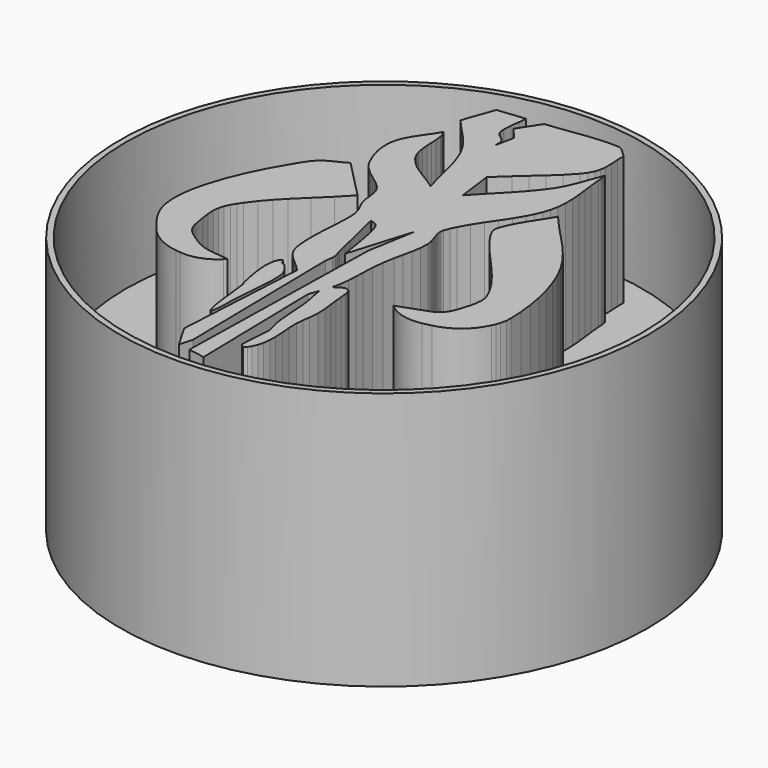
from build123d import *

# Parameters (mm, degrees)
F1_R     = 28.575
F2_DEPTH = 27.94
F0_R     = 27.94
F3_DEPTH = 13.97


# Not quite as in the source:
# - ends of sketch curves that miss each other by under 0.0002 mm in the source are joined


with BuildPart() as f2:
    # F1 (on face) → F2 (new body)
    with BuildSketch(Plane.XY):
        with Locations((1.0160021484, 3.1383140235)):
            Circle(F1_R)
    extrude(amount=-F2_DEPTH)

    # F0 (on Top) → F3 (cut)
    with BuildSketch(Plane.XY):
        with Locations((1.0160021484, 3.1383140235)):
            Circle(F0_R)
        Polygon((-3.3095653584, -5.6137892885), (-3.1695097584, -5.4395960885), (-3.0529237584, -5.4829538885), (-3.0004219584, -5.5103858885), (-2.9673765584, -5.5440408885), (-2.9427639584, -5.5983460885), (-2.9302163584, -5.6597632885), (-2.9131729584, -5.7589248885), (-2.8898557584, -5.8141190885), (-2.8479203584, -5.8575022885), (-2.7512733584, -5.9104104885), (-2.5523405584, -5.9840196885), (-2.5061633584, -6.0104102885), (-2.4849035584, -6.0263360885), (-2.4798235584, -6.0306286885), (-2.4773343584, -6.0328130885), (-2.4760897584, -6.0339306885), (-2.4754801584, -6.0344894885), (-2.4730163584, -6.0367246885), (-2.4632119584, -6.0456654885), (-2.4242229584, -6.0817588885), (-2.2726103584, -6.2308822885), (-1.9922197584, -6.5571706885), (-1.7587429584, -6.9181808885), (-1.5875723584, -7.3190944885), (-1.4959037584, -7.7449508885), (-1.4564575584, -8.7470316885), (-1.5075115584, -9.7528970885), (-1.5761169584, -10.7580258885), (-1.7809679584, -13.4732858885), (-1.8152833584, -14.2048566885), (-1.8169851584, -14.9385864885), (-1.8529515584, -15.6699794885), (-1.9431723584, -16.2117868885), (-1.9748207584, -16.3335290885), (-2.0227759584, -16.4506738885), (-2.0391081584, -16.4671838885), (-2.0507159584, -16.4732036885), (-2.0637969584, -16.4748800885), (-2.0751253584, -16.4723146885), (-2.0914321584, -16.4626372885), (-2.1228773584, -16.4262898885), (-2.1991789584, -16.2593356885), (-2.3008551584, -15.9096792885), (-2.3766995584, -15.5528854885), (-2.5239687584, -14.6005886885), (-2.6334681584, -13.6423736885), (-2.8588677584, -11.7314300885), (-2.9211739584, -11.2544434885), (-2.9539399584, -11.0161660885), (-2.9707801584, -10.8971162885), (-2.9752505584, -10.8818762885), (-2.9848009584, -10.8691762885), (-3.0330101584, -10.8370960885), (-3.0537111584, -10.8222878885), (-3.0650903584, -10.8089274885), (-3.0688241584, -10.8010026885), (-3.0700179584, -10.7968116885), (-3.0702465584, -10.7957448885), (-3.0703227584, -10.7954908885), (-3.0705259584, -10.7944240885), (-3.0713387584, -10.7901314885), (-3.0746661584, -10.7730372885), (-3.0882551584, -10.7046604885), (-3.1452781584, -10.4317374885), (-3.3700173584, -9.3393850885), (-3.4978301584, -8.5924472885), (-3.5894733584, -7.8403786885), (-3.6277003584, -7.0879798885), (-3.5682897584, -6.3395942885), (-3.5083711584, -6.0704558885), (-3.4161437584, -5.8112742885), align=None, mode=Mode.SUBTRACT)
        with BuildLine():
            Line((-10.3454923584, 11.6649163115), (-9.7154707584, 12.0162745115))
            Line((-9.7154707584, 12.0162745115), (-5.5498707584, 7.7514875115))
            Line((-5.5498707584, 7.7514875115), (-6.9198959584, 6.3156255115))
            Line((-6.9198959584, 6.3156255115), (-8.3367333584, 4.9403933115))
            Line((-8.3367333584, 4.9403933115), (-9.7384831584, 3.5689457115))
            Line((-9.7384831584, 3.5689457115), (-10.6222507584, 2.6428617115))
            Line((-10.6222507584, 2.6428617115), (-11.4586981584, 1.6763409115))
            Line((-11.4586981584, 1.6763409115), (-12.2270481584, 0.6563277115))
            Line((-12.2270481584, 0.6563277115), (-12.5530571584, 0.1778679115))
            Line((-12.5530571584, 0.1778679115), (-12.8566633584, -0.3166700885))
            Line((-12.8566633584, -0.3166700885), (-13.1114253584, -0.8399100885))
            Line((-13.1114253584, -0.8399100885), (-13.2776175584, -1.4147120885))
            Line((-13.2776175584, -1.4147120885), (-13.3395681584, -2.0160824885))
            Line((-13.3395681584, -2.0160824885), (-13.3030175584, -2.8127026885))
            Line((-13.3030175584, -2.8127026885), (-13.1902415584, -3.6027950885))
            Line((-13.1902415584, -3.6027950885), (-12.9876511584, -4.7950710885))
            ThreePointArc((-12.9876511584, -4.7950710885), (-12.6458886406, -5.7381027666), (-11.9657003768, -6.475296573))
            Line((-11.9657003768, -6.475296573), (-11.3262371584, -6.9315412885))
            Line((-11.3262371584, -6.9315412885), (-10.6611889584, -7.3559498885))
            Line((-10.6611889584, -7.3559498885), (-10.1669303584, -7.6130740885))
            Line((-10.1669303584, -7.6130740885), (-9.6479321584, -7.8141404885))
            Line((-9.6479321584, -7.8141404885), (-9.0811311584, -7.9525958885))
            Line((-9.0811311584, -7.9525958885), (-8.5008173584, -8.0379144885))
            Line((-8.5008173584, -8.0379144885), (-7.6721931584, -8.1176704885))
            Line((-7.6721931584, -8.1176704885), (-6.8392255584, -8.2166796885))
            Line((-6.8392255584, -8.2166796885), (-7.1013281584, -8.4787822885))
            ThreePointArc((-7.1013281584, -8.4787822885), (-8.7866271737, -9.5348586077), (-10.7637806827, -9.7502650449))
            Line((-10.7637806827, -9.7502650449), (-11.2680457584, -9.6909210885))
            ThreePointArc((-11.2680457584, -9.6909210885), (-13.3569404423, -9.0212773173), (-15.0397067215, -7.6140816273))
            Line((-15.0397067215, -7.6140816273), (-15.6487329584, -6.8493722885))
            Line((-15.6487329584, -6.8493722885), (-16.2212997584, -6.0557746885))
            Line((-16.2212997584, -6.0557746885), (-16.5837323584, -5.4619734885))
            Line((-16.5837323584, -5.4619734885), (-16.8932567584, -4.8286244885))
            Line((-16.8932567584, -4.8286244885), (-17.1266827584, -4.1564896885))
            Line((-17.1266827584, -4.1564896885), (-17.2765935584, -3.4465596885))
            Line((-17.2765935584, -3.4465596885), (-17.3543429584, -2.7171224885))
            Line((-17.3543429584, -2.7171224885), (-17.3680335584, -1.9835704885))
            Line((-17.3680335584, -1.9835704885), (-17.2836039584, -0.8674944885))
            Line((-17.2836039584, -0.8674944885), (-17.0950851584, 0.2349671115))
            Line((-17.0950851584, 0.2349671115), (-16.8279279584, 1.3131463115))
            Line((-16.8279279584, 1.3131463115), (-16.2564787584, 3.0786749115))
            Line((-16.2564787584, 3.0786749115), (-15.5659289584, 4.7901777115))
            Line((-15.5659289584, 4.7901777115), (-14.6148767584, 6.7561885115))
            Line((-14.6148767584, 6.7561885115), (-13.5328367584, 8.6467105115))
            Line((-13.5328367584, 8.6467105115), (-13.2243791584, 9.1616955115))
            Line((-13.2243791584, 9.1616955115), (-12.9099017584, 9.6756391115))
            Line((-12.9099017584, 9.6756391115), (-12.5667223584, 10.1631921115))
            Line((-12.5667223584, 10.1631921115), (-12.1721841584, 10.5990307115))
            Line((-12.1721841584, 10.5990307115), (-11.8060939584, 10.8919181115))
            Line((-11.8060939584, 10.8919181115), (-11.4065011584, 11.1371297115))
            Line((-11.4065011584, 11.1371297115), (-10.9902459584, 11.3523693115))
            Line((-10.9902459584, 11.3523693115), (-10.3454923584, 11.6649163115))
        make_face(mode=Mode.SUBTRACT)
        Polygon((8.0661040416, 22.4261343115), (8.5338704416, 23.6204931115), (8.5923920416, 23.3269199115), (8.6183762416, 23.1795237115), (8.6328542416, 23.0303495115), (8.6330320416, 23.0256759115), (8.6337686416, 23.0069815115), (8.6369182416, 22.9321785115), (8.6535298416, 22.6331443115), (8.7672202416, 21.4402841115), (8.8865494416, 20.4831359115), (9.0008240416, 19.5213649115), (9.0800466416, 18.5585525115), (9.0942960416, 17.5982801115), (9.0136510416, 16.6440783115), (8.8528182416, 15.8703435115), (8.6087496416, 15.1157857115), (8.2981838416, 14.3845705115), (7.9378594416, 13.6808635115), (7.3038500416, 12.6231059115), (6.6187358416, 11.5943551115), (5.9217598416, 10.5717511115), (5.2521396416, 9.5324847115), (4.6490674416, 8.4536959115), (4.3606504416, 7.8614949115), (4.1353270416, 7.2449861115), (4.0925788416, 6.9641129115), (4.1026118416, 6.6794043115), (4.1737572416, 6.3142539115), (4.2830534416, 5.9577649115), (4.4482042416, 5.4897191115), (4.5931874416, 5.0155011115), (4.6662124416, 4.5302087115), (4.6287728416, 3.5591413115), (4.4759664416, 2.5943477115), (4.2646130416, 1.6343293115), (4.0514562416, 0.6775875115), (3.8455384416, -0.5475052885), (3.7179542416, -1.7848408885), (3.6589754416, -3.0265960885), (3.6352772416, -3.9616462885), (3.5841724416, -4.8977124885), (3.4727934416, -5.8243806885), (3.2682218416, -6.7312368885), (3.4414752416, -6.6185370885), (3.5283686416, -6.5629110885), (3.5707612416, -6.5335232885), (3.5733774416, -6.5316436885), (3.5746728416, -6.5306784885), (3.5799052416, -6.5268938885), (3.6008348416, -6.5118316885), (3.6855692416, -6.4529798885), (4.0465286416, -6.2508466885), (4.2873714416, -6.1790154885), (4.4545034416, -6.1779740885), (4.5851610416, -6.2217382885), (4.6940762416, -6.3064980885), (4.8063442416, -6.4761446885), (4.8911802416, -6.7184860885), (4.9391100416, -6.9721812885), (5.0166562416, -7.7150550885), (5.0728664416, -8.4605704885), (5.1635952416, -9.2012852885), (5.2942782416, -10.2066934885), (5.3297366416, -11.2217536885), (5.2487614416, -12.2298542885), (5.1341820416, -13.0151714885), (5.0642558416, -13.8045526885), (5.0875984416, -14.8106212885), (5.1678370416, -15.8161056885), (5.2228026416, -16.8224536885), (5.2067498416, -17.5585964885), (5.1168084416, -18.2882368885), (4.9692344416, -18.8575778885), (4.7352242416, -19.3954228885), (4.5239978416, -19.7238702885), (4.2690834416, -20.0192468885), (4.0580856416, -19.8658054885), (3.9541234416, -19.7850080885), (3.8989800416, -19.7162756885), (3.8755612416, -19.6531312885), (3.8732244416, -19.6366466885), (3.8725894416, -19.6283662885), (3.8724116416, -19.6242260885), (3.8723608416, -19.6231846885), (3.8722592416, -19.6190190885), (3.8718274416, -19.6024074885), (3.8704558416, -19.5359102885), (3.8697954416, -19.2698960885), (3.9251420416, -18.2064742885), (4.0465540416, -16.7551944885), (4.0697696416, -16.3887740885), (4.0461222416, -16.0254270885), (3.9571714416, -15.6713764885), (3.8490182416, -15.3222534885), (3.6780762416, -14.5939846885), (3.5841724416, -13.8480882885), (3.5269716416, -13.0982548885), (3.3674088416, -10.8850766885), (3.2837920416, -10.1266326885), (3.1492482416, -9.3764690885), (3.0318748416, -8.8792132885), (2.9315194416, -8.3784522885), (2.8809226416, -7.8725096885), (2.4838190416, -9.0101248885), (2.7813546416, -23.4905886885), (0.9960902416, -23.1930276885), (1.4919998416, 0.4120813115), (2.3846320416, 5.5695005115), (0.3018320416, -1.2739960885), (0.0915962416, 0.0695877115), (-0.1240497584, 1.4122063115), (-0.3820375584, 2.7475605115), (-0.5009857584, 3.3255629115), (-0.6647141584, 3.8912463115), (-0.8834081584, 4.3707475115), (-1.0111701584, 4.5227411115), (-1.2562801584, 4.6632285115), (-1.5219895584, 4.7624409115), (-1.7809679584, 4.8752423115), (-0.8256231584, 0.8472595115), (-0.5964389584, -0.1624666885), (-0.3547833584, -1.1691702885), (-0.2221445584, -1.6122224885), (-0.1035011584, -2.0585512885), (-0.0757135584, -2.5098838885), (-0.1940775584, -3.2576090885), (0.1034580416, -21.6061372885), (-0.2932645584, -22.9946790885), (-1.7809679584, -20.4159694885), (-0.9875227584, -6.1338796885), (-1.4807907584, -5.6341092885), (-2.0100251584, -5.1712450885), (-2.5597827584, -4.6838952885), (-3.0595785584, -4.1487426885), (-3.3074317584, -3.7897898885), (-3.4946043584, -3.3963946885), (-3.6684419584, -2.7556034885), (-3.7596025584, -2.0930952885), (-3.8050431584, -1.4256848885), (-3.8107073584, 0.0444671115), (-3.7281065584, 1.5153049115), (-3.6398415584, 2.9859141115), (-3.6105553584, 3.7217013115), (-3.6112157584, 4.4578695115), (-3.6794909584, 5.1880179115), (-3.7738265584, 5.5503997115), (-3.9207401584, 5.8981511115), (-4.0918345584, 6.2345487115), (-4.2959743584, 6.6588811115), (-4.4605155584, 7.1009173115), (-4.5651635584, 7.5582697115), (-4.6428367584, 8.2881133115), (-4.7504565584, 9.0121149115), (-4.8538599584, 9.3518399115), (-5.0104255584, 9.6688065115), (-5.2961247584, 10.0398243115), (-5.6347829584, 10.3630901115), (-6.1587595584, 10.7813519115), (-6.7016083584, 11.1859485115), (-7.2371673584, 11.5971491115), (-7.7392491584, 12.0351721115), (-8.1817171584, 12.5202613115), (-8.5384093584, 13.0726605115), (-8.9882687584, 14.0837075115), (-9.3054893584, 15.1465451115), (-9.4336069584, 15.9750931115), (-9.4430303584, 16.8133439115), (-9.3338611584, 17.5000329115), (-9.1114079584, 18.1563181115), (-8.6753153584, 18.9827579115), (-8.1585523584, 19.7639603115), (-7.6245427584, 20.5370855115), (-7.1367611584, 21.3393191115), (-6.9672161584, 21.0473969115), (-6.8895937584, 20.8973845115), (-6.8592407584, 20.8183397115), (-6.8472011584, 20.7777251115), (-6.8420957584, 20.7571765115), (-6.8397843584, 20.7468387115), (-6.8392255584, 20.7442479115), (-6.8370411584, 20.7338847115), (-6.8285321584, 20.6923557115), (-6.7977981584, 20.5255285115), (-6.7172547584, 19.8507013115), (-6.6781387584, 19.1706163115), (-6.6455251584, 18.4886771115), (-6.5838539584, 17.8118941115), (-6.4574889584, 17.1472777115), (-6.2646013584, 16.5940657115), (-5.9806547584, 16.0841861115), (-5.4611993584, 15.4630291115), (-4.8518533584, 14.9281305115), (-4.1021977584, 14.4026553115), (-3.3204365584, 13.9190393115), (-2.5366433584, 13.4351693115), (-1.7809679584, 12.9089067115), (-2.2346119584, 14.6381387115), (-2.6529245584, 16.3778355115), (-2.9137317584, 17.3361521115), (-3.2208431584, 18.2799907115), (-3.6013097584, 19.2175301115), (-4.0769247584, 20.1075715115), (-4.5533017584, 20.7934985115), (-5.0823583584, 21.4401063115), (-5.6411837584, 22.0585709115), (-6.5040725584, 22.9759681115), (-7.3351097584, 23.9180287115), (-6.1449419584, 27.2901835115), (-3.1695097584, 27.5877191115), (-3.2667409584, 26.7103777115), (-3.3875941584, 25.8349667115), (-3.4357779584, 24.9566855115), (-3.3797963584, 24.3776417115), (-3.2721765584, 24.0808427115), (-3.1520091584, 23.9295349115), (-3.0097437584, 23.7978613115), (-2.6839125584, 23.5469601115), (-2.3816525584, 23.2716749115), (-2.2410635584, 23.0499329115), (-2.1877997584, 22.7911323115), (-2.1856915584, 22.5112751115), (-2.1776905584, 22.2319513115), (-1.7809679584, 24.2155643115), (-2.8719741584, 25.5049191115), (-1.3842453584, 27.7860931115), (0.5081562416, 28.0123817115), (2.3984242416, 28.2699377115), (3.3428470416, 28.3786751115), (4.2880572416, 28.4573897115), (5.2325054416, 28.4933815115), (5.9890698416, 28.4830945115), (6.1937684416, 28.4589391115), (6.3889166416, 28.3953375115), (6.6050706416, 28.2646799115), (6.7997362416, 28.1014849115), (7.1619402416, 27.7336167115), (7.5420512416, 27.3893705115), (7.5523890416, 26.5162455115), (7.6090818416, 25.6425363115), (7.6128410416, 24.7698177115), (7.5422290416, 24.2320743115), (7.3854094416, 23.7152351115), (7.0637184416, 23.1157189115), (6.6520098416, 22.5731495115), (5.6734494416, 21.5312669115), (4.6261312416, 20.5515127115), (3.5477488416, 19.5987079115), (2.4760212416, 18.6376481115), (0.8969286416, 17.1737191115), (1.3928128416, 13.3056293115), (2.7371586416, 14.7357255115), (4.1018752416, 16.1440285115), (4.9437836416, 17.0521039115), (5.7479984416, 17.9923611115), (6.4934884416, 18.9767127115), (6.9340006416, 19.6884715115), (7.3056534416, 20.4422673115), (7.6250330416, 21.2196851115), align=None, mode=Mode.SUBTRACT)
        with BuildLine():
            ThreePointArc((13.3561343411, -7.132521402), (11.3316611954, -7.1213781471), (9.5221088802, -6.2135587222))
            Line((9.5221088802, -6.2135587222), (9.4265026416, -6.1338796885))
            Line((9.4265026416, -6.1338796885), (12.5173270416, -5.0099296885))
            ThreePointArc((12.5173270416, -5.0099296885), (13.4896977223, -4.3734525934), (14.0767872311, -3.3704872396))
            Line((14.0767872311, -3.3704872396), (14.1046746416, -3.2805706885))
            Line((14.1046746416, -3.2805706885), (14.3008134416, -2.6644682885))
            Line((14.3008134416, -2.6644682885), (14.4844808416, -2.0442256885))
            Line((14.4844808416, -2.0442256885), (14.6265176416, -1.4026724885))
            Line((14.6265176416, -1.4026724885), (14.6799846416, -0.7477334885))
            Line((14.6799846416, -0.7477334885), (14.6443738416, -0.3363042885))
            Line((14.6443738416, -0.3363042885), (14.5441200416, 0.0614851115))
            Line((14.5441200416, 0.0614851115), (14.2042172416, 0.8476659115))
            Line((14.2042172416, 0.8476659115), (13.7782338416, 1.5889649115))
            Line((13.7782338416, 1.5889649115), (13.3048032416, 2.2973963115))
            Line((13.3048032416, 2.2973963115), (12.5176064416, 3.3441811115))
            Line((12.5176064416, 3.3441811115), (11.6722436416, 4.3474049115))
            Line((11.6722436416, 4.3474049115), (10.7968326416, 5.3292419115))
            Line((10.7968326416, 5.3292419115), (9.4878436416, 6.8087919115))
            Line((9.4878436416, 6.8087919115), (8.4190370416, 8.1488451115))
            Line((8.4190370416, 8.1488451115), (7.9258706416, 8.8534157115))
            Line((7.9258706416, 8.8534157115), (7.6935114416, 9.2257289115))
            Line((7.6935114416, 9.2257289115), (7.5055514416, 9.6219943115))
            Line((7.5055514416, 9.6219943115), (7.4370730416, 9.8464033115))
            Line((7.4370730416, 9.8464033115), (7.4034180416, 10.0783561115))
            Line((7.4034180416, 10.0783561115), (7.4201312416, 10.3152111115))
            Line((7.4201312416, 10.3152111115), (7.4785512416, 10.5465797115))
            Line((7.4785512416, 10.5465797115), (7.7880756416, 11.3548839115))
            Line((7.7880756416, 11.3548839115), (8.1760606416, 12.1276789115))
            Line((8.1760606416, 12.1276789115), (8.8142864416, 13.1896275115))
            Line((8.8142864416, 13.1896275115), (9.4846940416, 14.2297575115))
            Line((9.4846940416, 14.2297575115), (10.1207608416, 15.2892677115))
            Line((10.1207608416, 15.2892677115), (11.3126304416, 13.9281579115))
            Line((11.3126304416, 13.9281579115), (12.5453432416, 12.6205913115))
            Line((12.5453432416, 12.6205913115), (13.7624604416, 11.3159203115))
            Line((13.7624604416, 11.3159203115), (14.6354330416, 10.2954499115))
            Line((14.6354330416, 10.2954499115), (15.4457184416, 9.2193535115))
            Line((15.4457184416, 9.2193535115), (16.1708122416, 8.0821193115))
            Line((16.1708122416, 8.0821193115), (16.7882354416, 6.8782863115))
            Line((16.7882354416, 6.8782863115), (17.3346656416, 5.5204023115))
            Line((17.3346656416, 5.5204023115), (17.7829756416, 4.1131661115))
            Line((17.7829756416, 4.1131661115), (18.1356546416, 2.6702175115))
            Line((18.1356546416, 2.6702175115), (18.3951410416, 1.2052471115))
            Line((18.3951410416, 1.2052471115), (18.5628318416, -0.2451436885))
            Line((18.5628318416, -0.2451436885), (18.6484298416, -1.7055674885))
            Line((18.6484298416, -1.7055674885), (18.6148510416, -2.3249464885))
            Line((18.6148510416, -2.3249464885), (18.4841680416, -2.9266724885))
            Line((18.4841680416, -2.9266724885), (18.3346636416, -3.3551958885))
            Line((18.3346636416, -3.3551958885), (18.1562032416, -3.7687078885))
            ThreePointArc((18.1562032416, -3.7687078885), (16.5671418558, -5.8024333082), (14.2454107654, -6.9296893542))
            Line((14.2454107654, -6.9296893542), (13.3561343411, -7.132521402))
        make_face(mode=Mode.SUBTRACT)
    extrude(amount=-F3_DEPTH, mode=Mode.SUBTRACT)


solid = f2.part
